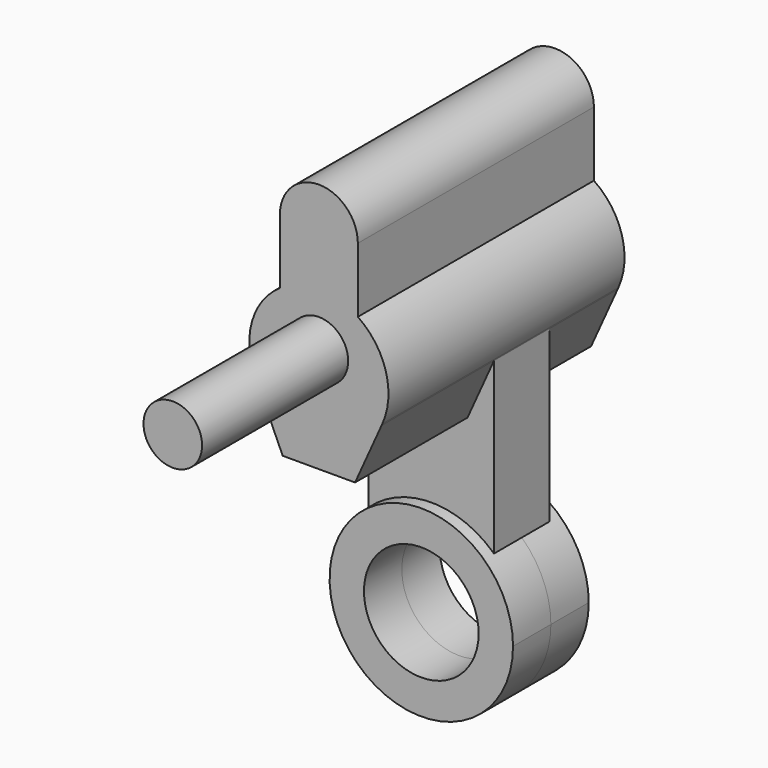
from build123d import *

# Parameters (mm, degrees)
F0_R     = 20.6
F1_DEPTH = 17
F2_DEPTH = 12.5
F4_DEPTH = 43
F5_DEPTH = 20
F6_R     = 10.5222684304
F7_DEPTH = 65.6


# Not quite as in the source:
# - a feature names something its author has since deleted; it is built from what else it names


with BuildPart() as f1:
    # F0 (on Front) → F1 (new body, symmetric)
    with BuildSketch(Plane.XZ):
        with BuildLine():
            ThreePointArc((-22.5, 24.0694217363), (-13.1196699102, -30.2235226962), (32.9482482496, 0))
            ThreePointArc((32.9482482496, 0), (30.2235226962, 13.1196699102), (22.5, 24.0694217363))
            ThreePointArc((22.5, 24.0694217363), (0, 32.9482482496), (-22.5, 24.0694217363))
        make_face()
        Circle(F0_R, mode=Mode.SUBTRACT)
    extrude(amount=F1_DEPTH, both=True)

    # F0 (on Front) → F2 (join, symmetric)
    with BuildSketch(Plane.XZ):
        with BuildLine():
            ThreePointArc((-22.5, 24.0694217363), (0, 32.9482482496), (22.5, 24.0694217363))
            Line((22.5, 24.0694217363), (22.5, 85.0795575915))
            Line((22.5, 85.0795575915), (13, 64))
            Line((13, 64), (-13, 64))
            Line((-13, 64), (-22.5, 85.0795575915))
            Line((-22.5, 85.0795575915), (-22.5, 24.0694217363))
        make_face()
        Polygon((13, 64), (22.5, 85.0795575915), (22.5, 96), (-22.5, 96), (-22.5, 85.0795575915), (-13, 64), align=None)
    extrude(amount=F2_DEPTH, both=True)


with BuildPart() as f4:
    # F3 (on Front) → F4 (new body, symmetric)
    with BuildSketch(Plane.XZ):
        with BuildLine():
            Line((13, 64), (22.5, 85.0795575915))
            Line((22.5, 85.0795575915), (22.7922887347, 85.7281172985))
            ThreePointArc((22.7922887347, 85.7281172985), (24.0504315373, 102.8247155888), (14, 116.7123151772))
            Line((14, 116.7123151772), (14, 140))
            ThreePointArc((14, 140), (0, 154), (-14, 140))
            Line((-14, 140), (-14, 116.7123151772))
            ThreePointArc((-14, 116.7123151772), (-24.0504315373, 102.8247155888), (-22.7922887347, 85.7281172985))
            Line((-22.7922887347, 85.7281172985), (-22.5, 85.0795575915))
            Line((-22.5, 85.0795575915), (-13, 64))
            Line((-13, 64), (13, 64))
        make_face()
    extrude(amount=F4_DEPTH, both=True)

    # F5 (add): a face of the model
    f5_faces = [f4.faces().sort_by_distance(p)[0] for p in [
        (0, -43, 104.5669509918),
    ]]
    extrude(f5_faces, amount=F5_DEPTH)

    # F6 (on face) → F7 (join)
    with BuildSketch(Plane.XZ.offset(63)):
        with Locations((0, 101.6081124544)):
            Circle(F6_R)
    extrude(amount=F7_DEPTH)


solid = Compound([f1.part, f4.part])
